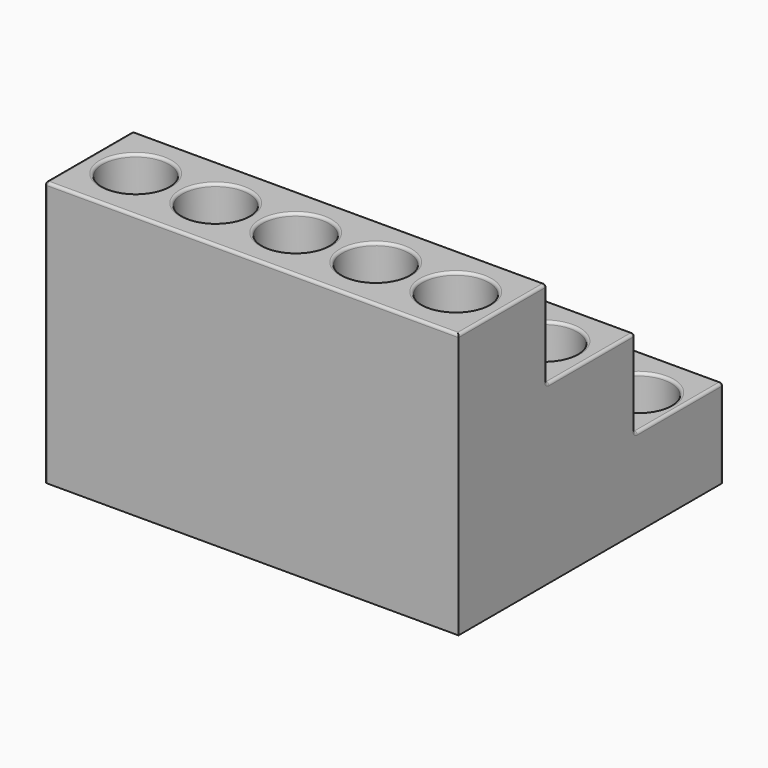
from build123d import *

# Parameters (mm, degrees)
F1_DEPTH = 150
F2_R     = 12
F3_R     = 12
F4_DEPTH = 30
F5_R     = 12
F5_R_2   = 8.5
F6_DEPTH = 30
F7_R     = 0.99999


# Not quite as in the source:
# - a fillet or chamfer is up to 0.001 mm smaller than in the source, because OpenCascade refuses the exact size


with BuildPart() as f1:
    # F0 (on Right) → F1 (new body)
    with BuildSketch(Plane.YZ):
        Polygon((0, 96), (0, 0), (120, 0), (120, 32), (80, 32), (80, 64), (40, 64), (40, 96), align=None)
    extrude(amount=F1_DEPTH)

    # F2 (on face) + F3 (on face) → F4 (cut)
    with BuildSketch(Plane.XY.offset(96)):
        with Locations((133, 20)):
            Circle(F2_R)
        with Locations((104, 20)):
            Circle(F2_R)
        with Locations((75, 20)):
            Circle(F2_R)
        with Locations((46, 20)):
            Circle(F2_R)
        with Locations((17, 20)):
            Circle(F2_R)
    with BuildSketch(Plane.XY.offset(64)):
        with Locations((17, 60)):
            Circle(F3_R)
        with Locations((46, 60)):
            Circle(F3_R)
        with Locations((75, 60)):
            Circle(F3_R)
        with Locations((104, 60)):
            Circle(F3_R)
        with Locations((133, 60)):
            Circle(F3_R)
    extrude(amount=-F4_DEPTH, mode=Mode.SUBTRACT)

    # F5 (on face) → F6 (cut)
    with BuildSketch(Plane.XY.offset(32)):
        with Locations((135, 100)):
            Circle(F5_R)
        with Locations((109, 100)):
            Circle(F5_R)
        with Locations((83, 100)):
            Circle(F5_R)
        with Locations((57, 100)):
            Circle(F5_R)
        with Locations((31, 100)):
            Circle(F5_R)
        with Locations((10.5, 90.5)):
            Circle(F5_R_2)
        with Locations((10.5, 109.5)):
            Circle(F5_R_2)
    extrude(amount=-F6_DEPTH, mode=Mode.SUBTRACT)

    # F7 (radius 1 in the source; OpenCascade refuses exactly that, so slightly less here)
    f7_edges = [f1.edges().sort_by_distance(p)[0] for p in [
        (75, 0, 96),
        (150, 20, 96),
        (75, 40, 96),
        (0, 20, 96),
        (5, 20, 96),
        (34, 20, 96),
        (63, 20, 96),
        (92, 20, 96),
        (121, 20, 96),
        (150, 40, 80),
        (150, 60, 64),
        (150, 80, 48),
        (75, 80, 64),
        (75, 40, 64),
        (0, 40, 80),
        (0, 60, 64),
        (5, 60, 64),
        (34, 60, 64),
        (63, 60, 64),
        (92, 60, 64),
        (121, 60, 64),
        (0, 80, 48),
        (0, 0, 48),
        (0, 120, 16),
        (150, 120, 16),
        (150, 100, 32),
        (75, 80, 32),
        (123, 100, 32),
        (97, 100, 32),
        (95, 100, 17),
        (71, 100, 32),
        (71, 100, 2),
        (75, 120, 32),
        (45, 100, 32),
        (19, 100, 32),
        (123, 100, 2),
        (97, 100, 2),
        (19, 100, 2),
        (2, 90.5, 2),
        (2, 109.5, 2),
        (5, 60, 34),
        (34, 60, 34),
        (63, 60, 34),
        (92, 60, 34),
        (121, 60, 34),
        (5, 20, 66),
        (34, 20, 66),
        (63, 20, 66),
        (92, 20, 66),
        (121, 20, 66),
        (0, 100, 32),
    ]]
    fillet(f7_edges, radius=F7_R)


solid = f1.part
